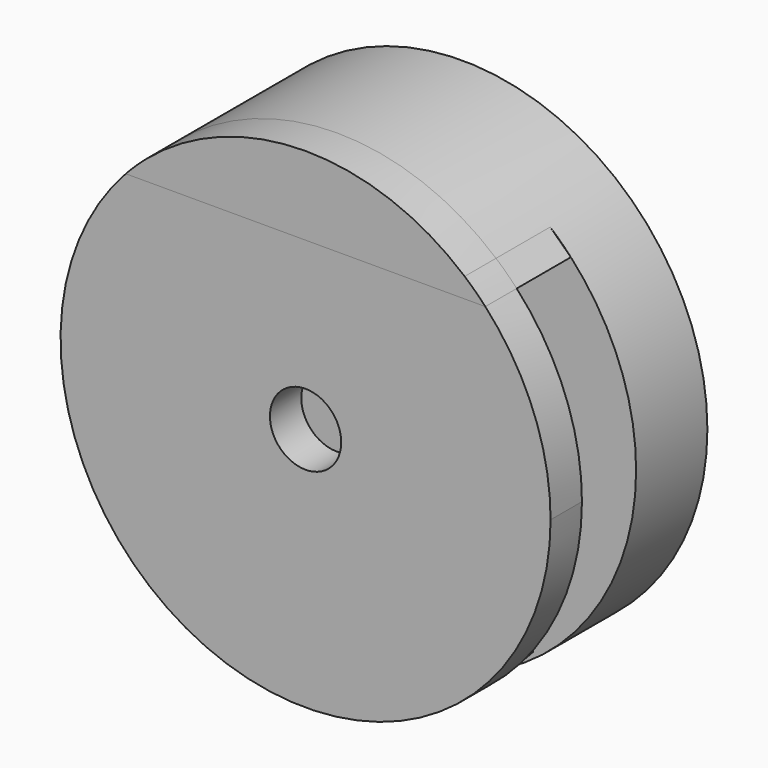
from build123d import *

# Parameters (mm, degrees)
F0_R         = 34.925
F1_DEPTH     = 12.7
F2_R         = 5.08
F3_DEPTH     = 6.35
F5_DEPTH     = 15.24
F6_DEPTH     = 15.24
F7_R         = 34.925
F8_DEPTH     = 5.588
F9_R         = 5.08
F10_DEPTH    = 6.35
F13_DEPTH    = 2.54
F14_T1_DEPTH = 60.8716457984
F15_DEPTH    = 2.54
F16_R        = 2.53999
F17_R        = 3.175
F18_DEPTH    = 25.4


# Not quite as in the source:
# - a fillet or chamfer that OpenCascade refuses, or shapes differently, is made with other operations: its cross-section is extruded or revolved along the edge and cut away or added
# - a fillet or chamfer is up to 0.001 mm smaller than in the source, because OpenCascade refuses the exact size


with BuildPart() as f1:
    # F0 (on Front) → F1 (new body)
    with BuildSketch(Plane.XZ):
        Circle(F0_R)
    extrude(amount=F1_DEPTH)

    # F2 (on face) → F3 (cut)
    with BuildSketch(Plane.XZ.offset(12.7)):
        Circle(F2_R)
    extrude(amount=-F3_DEPTH, mode=Mode.SUBTRACT)

    # F4 (on face) → F5 (join)
    with BuildSketch(Plane.XZ.offset(12.7)):
        Polygon((22.6792097043, 26.5595382526), (-22.6792097043, 26.5595382526), (-25.6262624144, 23.7286809509), (25.6262624144, 23.7286809509), align=None)
    extrude(amount=F5_DEPTH)

    # F6 (add): a face of the model
    f6_faces = [f1.faces().sort_by_distance(p)[0] for p in [
        (0, -12.7, 29.942642138),
    ]]
    extrude(f6_faces, amount=F6_DEPTH)

    # F7 (on face) → F8 (join)
    with BuildSketch(Plane.XZ.offset(27.94)):
        Circle(F7_R)
    extrude(amount=-F8_DEPTH)

    # F9 (on face) → F10 (cut)
    with BuildSketch(Plane.XZ.offset(27.94)):
        Circle(F9_R)
    extrude(amount=-F10_DEPTH, mode=Mode.SUBTRACT)

    # F12 (on face) → F13 (join)
    with BuildSketch(Plane(origin=(0, -22.352, 0), x_dir=(-1, 0, 0), z_dir=(0, 1, 0))):
        Polygon((-25.9485930492, -22.8007244613), (-24.3002702047, -24.7332440084), (24.2399447162, -24.7332440084), (25.8882675608, -22.8007244613), align=None)
    extrude(amount=F13_DEPTH)

    # F14: fillet of radius 2.54 on 1 edges, made by hand

    # F14_s2 → F14_t1 (cut)
    with BuildSketch(Plane.YZ.offset(-30.405660155)):
        with BuildLine():
            ThreePointArc((-22.2782861755, -24.7332440084), (-20.7116656647, -24.1925689383), (-19.812, -22.8007244613))
            Line((-19.812, -22.8007244613), (-19.812, -24.7332440084))
            Line((-19.812, -24.7332440084), (-22.2782861755, -24.7332440084))
        make_face()
    extrude(amount=F14_T1_DEPTH, mode=Mode.SUBTRACT)

    # F15 (add): a face of the model
    f15_faces = [f1.faces().sort_by_distance(p)[0] for p in [
        (0.0301627442, -21.082, -22.8007244613),
    ]]
    extrude(f15_faces, amount=F15_DEPTH)

    # F16 (radius 2.54 in the source; OpenCascade refuses exactly that, so slightly less here)
    f16_edges = [f1.edges().sort_by_distance(p)[0] for p in [
        (0.030163, -19.812, -20.260724),
    ]]
    fillet(f16_edges, radius=F16_R)

    # F17 (on face) → F18 (cut)
    with BuildSketch(Plane(origin=(0, -22.352, 0), x_dir=(-1, 0, 0), z_dir=(0, 1, 0))):
        Circle(F17_R)
    extrude(amount=F18_DEPTH, mode=Mode.SUBTRACT)


solid = f1.part
